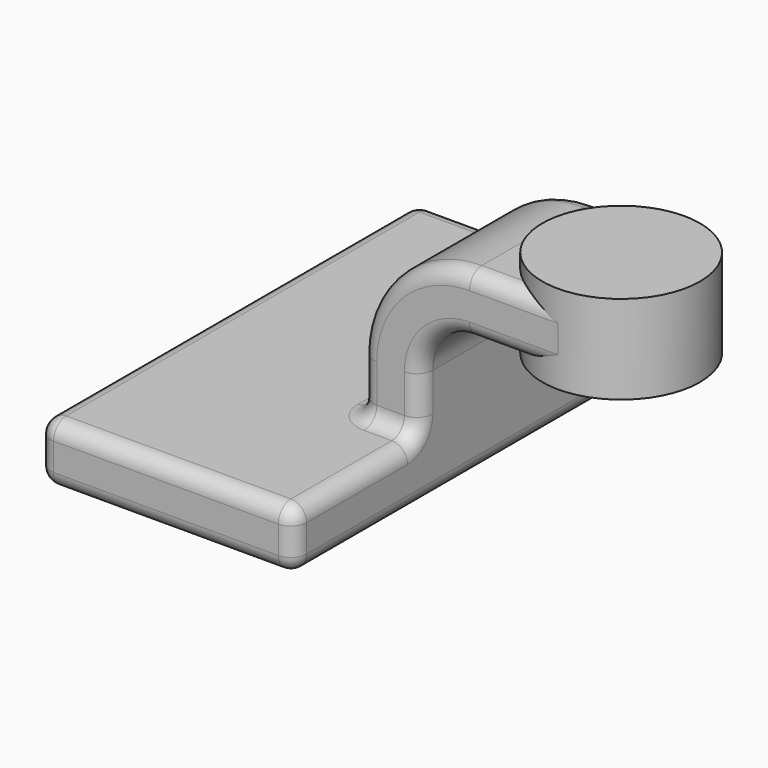
from build123d import *

# Parameters (mm, degrees)
F1_DEPTH      = 76.2
F0_W          = 25.4
F0_H          = 19.05
F2_DEPTH      = 25.4
F4_T1_DEPTH   = 142.24
F4_T3_DEPTH   = 90.17
F4_T5_DEPTH   = 17.4752
F4_T7_DEPTH   = 72.39
F4_T9_DEPTH   = 26.67
F4_T11_DEPTH  = 8.89
F4_S15_W      = 5.1816
F4_S15_H      = 5.1816
F4_T16_DEPTH  = 5.1816
F4_S21_W      = 5.1816
F4_S21_H      = 5.1816
F4_T22_DEPTH  = 5.1816
F4_S27_W      = 5.1816
F4_S27_H      = 5.1816
F4_T28_DEPTH  = 5.1816
F4_S33_W      = 5.1816
F4_S33_H      = 5.1816
F4_T34_DEPTH  = 5.1816
F4_S39_W      = 5.1816
F4_S39_H      = 5.1816
F4_T40_DEPTH  = 5.1816
F4_S45_W      = 5.1816
F4_S45_H      = 5.1816
F4_T46_DEPTH  = 5.1816
F4_T50_ANGLE  = 90
F4_T54_DEPTH  = 50.165
F4_S55_R      = 25.4
F4_T56_DEPTH  = 27
F4_T58_ANGLE  = 90
F4_T62_DEPTH  = 50.165
F4_S63_R      = 25.4
F4_T64_DEPTH  = 27
F4_T65_DEPTH  = 13.97
F4_T67_DEPTH  = 40.64
F4_T70_ANGLE  = 90
F4_T72_ANGLE  = 90
F4_T73_DEPTH  = 40.64
F4_T75_DEPTH  = 40.64
F4_T77_DEPTH  = 12.3952
F4_S81_W      = 5.1816
F4_S81_H      = 5.1816
F4_T82_DEPTH  = 5.1816
F4_S87_W      = 5.1816
F4_S87_H      = 5.1816
F4_T88_DEPTH  = 5.1816
F4_T92_ANGLE  = 90
F4_T96_DEPTH  = 50.165
F4_S97_R      = 25.4
F4_T98_DEPTH  = 27
F4_T100_ANGLE = 90
F4_T104_DEPTH = 50.165
F4_S105_R     = 25.4
F4_T106_DEPTH = 27
F4_T108_ANGLE = 90
F4_T110_ANGLE = 90


# Not quite as in the source:
# - a fillet or chamfer that OpenCascade refuses, or shapes differently, is made with other operations: its cross-section is extruded or revolved along the edge and cut away or added


with BuildPart() as f1:
    # F0 (on Front) → F1 (new body, symmetric)
    with BuildSketch(Plane.XZ):
        Polygon((-41.275, -9.525), (41.275, -9.525), (41.275, 9.525), (22.225, 9.525), (-41.275, 9.525), align=None)
    extrude(amount=F1_DEPTH, both=True)

    # F0 (on Front) → F2 (join, symmetric)
    with BuildSketch(Plane.XZ):
        with BuildLine():
            Line((22.225, 9.525), (41.275, 9.525))
            Line((41.275, 9.525), (41.275, 27.0002))
            ThreePointArc((41.275, 27.0002), (45.9246798487, 38.2255201513), (57.15, 42.8752))
            Line((57.15, 42.8752), (60.325, 42.8752))
            Line((60.325, 42.8752), (60.325, 61.9252))
            Line((60.325, 61.9252), (57.15, 61.9252))
            ThreePointArc((57.15, 61.9252), (32.4542956671, 51.6959043329), (22.225, 27.0002))
            Line((22.225, 27.0002), (22.225, 9.525))
        make_face()
        with Locations((73.025, 52.4002)):
            Rectangle(F0_W, F0_H)
    extrude(amount=F2_DEPTH, both=True)

    # F0 (on Front) → F3 (revolve)
    with BuildSketch(Plane.XZ):
        Polygon((85.725, 61.9252), (85.725, 42.8752), (85.725, 38.1), (111.125, 38.1), (111.125, 66.675), (85.725, 66.675), align=None)
    revolve(axis=Axis((85.725, 0, 52.3875), (0, 0, 1)))

    # F4: fillet of radius 5.08 on 31 edges, made by hand

    # F4_s2 → F4_t1 (cut)
    with BuildSketch(Plane.XZ.offset(-71.12)):
        with BuildLine():
            ThreePointArc((-41.275, 4.445), (-39.7871024484, 8.0371024484), (-36.195, 9.525))
            Line((-36.195, 9.525), (-41.275, 9.525))
            Line((-41.275, 9.525), (-41.275, 4.445))
        make_face()
        with BuildLine():
            ThreePointArc((-36.195, -9.525), (-39.7871024484, -8.0371024484), (-41.275, -4.445))
            Line((-41.275, -4.445), (-41.275, -9.525))
            Line((-41.275, -9.525), (-36.195, -9.525))
        make_face()
        with BuildLine():
            ThreePointArc((36.195, -9.525), (39.7871024484, -8.0371024484), (41.275, -4.445))
            Line((41.275, -4.445), (41.275, -9.525))
            Line((41.275, -9.525), (36.195, -9.525))
        make_face()
    extrude(amount=F4_T1_DEPTH, mode=Mode.SUBTRACT)

    # F4_s4 → F4_t3 (cut)
    with BuildSketch(Plane.YZ.offset(-36.195)):
        with BuildLine():
            ThreePointArc((76.2, 4.445), (74.7121024484, 8.0371024484), (71.12, 9.525))
            Line((71.12, 9.525), (76.2, 9.525))
            Line((76.2, 9.525), (76.2, 4.445))
        make_face()
        with BuildLine():
            ThreePointArc((-76.2, 4.445), (-74.7121024484, 8.0371024484), (-71.12, 9.525))
            Line((-71.12, 9.525), (-76.2, 9.525))
            Line((-76.2, 9.525), (-76.2, 4.445))
        make_face()
    extrude(amount=F4_T3_DEPTH, mode=Mode.SUBTRACT)

    # F4_s6 → F4_t5 (cut)
    with BuildSketch(Plane.XY.offset(9.525)):
        with BuildLine():
            ThreePointArc((27.305, -25.4), (23.7128975516, -23.9121024484), (22.225, -20.32))
            Line((22.225, -20.32), (22.225, -25.4))
            Line((22.225, -25.4), (27.305, -25.4))
        make_face()
        with BuildLine():
            ThreePointArc((27.305, 25.4), (23.7128975516, 23.9121024484), (22.225, 20.32))
            Line((22.225, 20.32), (22.225, 25.4))
            Line((22.225, 25.4), (27.305, 25.4))
        make_face()
    extrude(amount=F4_T5_DEPTH, mode=Mode.SUBTRACT)

    # F4_s8 → F4_t7 (cut)
    with BuildSketch(Plane.YZ.offset(-36.195)):
        with BuildLine():
            ThreePointArc((71.12, -9.525), (74.7121024484, -8.0371024484), (76.2, -4.445))
            Line((76.2, -4.445), (76.2, -9.525))
            Line((76.2, -9.525), (71.12, -9.525))
        make_face()
        with BuildLine():
            ThreePointArc((-71.12, -9.525), (-74.7121024484, -8.0371024484), (-76.2, -4.445))
            Line((-76.2, -4.445), (-76.2, -9.525))
            Line((-76.2, -9.525), (-71.12, -9.525))
        make_face()
    extrude(amount=F4_T7_DEPTH, mode=Mode.SUBTRACT)

    # F4_s10 → F4_t9 (cut)
    with BuildSketch(Plane.XY.offset(-4.445)):
        with BuildLine():
            ThreePointArc((36.195, 76.2), (39.7871024484, 74.7121024484), (41.275, 71.12))
            Line((41.275, 71.12), (41.275, 76.2))
            Line((41.275, 76.2), (36.195, 76.2))
        make_face()
        with BuildLine():
            ThreePointArc((41.275, -71.12), (39.7871024484, -74.7121024484), (36.195, -76.2))
            Line((36.195, -76.2), (41.275, -76.2))
            Line((41.275, -76.2), (41.275, -71.12))
        make_face()
    extrude(amount=F4_T9_DEPTH, mode=Mode.SUBTRACT)

    # F4_s12 → F4_t11 (cut)
    with BuildSketch(Plane.XY.offset(-4.445)):
        with BuildLine():
            ThreePointArc((-36.195, 76.2), (-39.7871024484, 74.7121024484), (-41.275, 71.12))
            Line((-41.275, 71.12), (-41.275, 76.2))
            Line((-41.275, 76.2), (-36.195, 76.2))
        make_face()
        with BuildLine():
            ThreePointArc((-36.195, -76.2), (-39.7871024484, -74.7121024484), (-41.275, -71.12))
            Line((-41.275, -71.12), (-41.275, -76.2))
            Line((-41.275, -76.2), (-36.195, -76.2))
        make_face()
    extrude(amount=F4_T11_DEPTH, mode=Mode.SUBTRACT)


with BuildPart() as f4_tool14:
    # F4_s15 → F4_t16 (new body)
    with BuildSketch(Plane.XZ.offset(71.12)):
        with Locations((-38.7858, 7.0358)):
            Rectangle(F4_S15_W, F4_S15_H)
    extrude(amount=F4_T16_DEPTH)

    # F4_s17 → F4_t18 (revolve, cut)
    with BuildSketch(Plane(origin=(-36.195, -71.12, 4.445), x_dir=(0.7071067812, 0, -0.7071067812), z_dir=(-0.7071067812, 0, -0.7071067812))):
        with BuildLine():
            ThreePointArc((0, -5.08), (5.08, 0), (0, 5.08))
            Line((0, 5.08), (0, -5.08))
        make_face()
    revolve(axis=Axis((-36.195, -71.12, 4.445), (0, -1, 0)), mode=Mode.SUBTRACT)


with BuildPart() as f1_1:
    add(f1.part)

    # F4_t13: cut F4_tool14
    add(f4_tool14.part, mode=Mode.SUBTRACT)


with BuildPart() as f4_tool20:
    # F4_s21 → F4_t22 (new body)
    with BuildSketch(Plane.XZ.offset(-71.12)):
        with Locations((-38.7858, 7.0358)):
            Rectangle(F4_S21_W, F4_S21_H)
    extrude(amount=-F4_T22_DEPTH)

    # F4_s23 → F4_t24 (revolve, cut)
    with BuildSketch(Plane(origin=(-36.195, 71.12, 4.445), x_dir=(0.7071067812, 0, -0.7071067812), z_dir=(0.7071067812, 0, 0.7071067812))):
        with BuildLine():
            ThreePointArc((0, -5.08), (5.08, 0), (0, 5.08))
            Line((0, 5.08), (0, -5.08))
        make_face()
    revolve(axis=Axis((-36.195, 71.12, 4.445), (0, 1, 0)), mode=Mode.SUBTRACT)


with BuildPart() as f1_2:
    add(f1_1.part)

    # F4_t19: cut F4_tool20
    add(f4_tool20.part, mode=Mode.SUBTRACT)


with BuildPart() as f4_tool26:
    # F4_s27 → F4_t28 (new body)
    with BuildSketch(Plane.XY.offset(-4.445)):
        with Locations((-38.7858, 73.7108)):
            Rectangle(F4_S27_W, F4_S27_H)
    extrude(amount=-F4_T28_DEPTH)

    # F4_s29 → F4_t30 (revolve, cut)
    with BuildSketch(Plane(origin=(-36.195, 71.12, -4.445), x_dir=(0.7071067812, -0.7071067812, 0), z_dir=(0.7071067812, 0.7071067812, 0))):
        with BuildLine():
            ThreePointArc((0, -5.08), (5.08, 0), (0, 5.08))
            Line((0, 5.08), (0, -5.08))
        make_face()
    revolve(axis=Axis((-36.195, 71.12, -4.445), (0, 0, -1)), mode=Mode.SUBTRACT)


with BuildPart() as f1_3:
    add(f1_2.part)

    # F4_t25: cut F4_tool26
    add(f4_tool26.part, mode=Mode.SUBTRACT)


with BuildPart() as f4_tool32:
    # F4_s33 → F4_t34 (new body)
    with BuildSketch(Plane.XY.offset(-4.445)):
        with Locations((38.7858, 73.7108)):
            Rectangle(F4_S33_W, F4_S33_H)
    extrude(amount=-F4_T34_DEPTH)

    # F4_s35 → F4_t36 (revolve, cut)
    with BuildSketch(Plane(origin=(36.195, 71.12, -4.445), x_dir=(-0.7071067812, -0.7071067812, 0), z_dir=(0.7071067812, -0.7071067812, 0))):
        with BuildLine():
            ThreePointArc((0, -5.08), (5.08, 0), (0, 5.08))
            Line((0, 5.08), (0, -5.08))
        make_face()
    revolve(axis=Axis((36.195, 71.12, -4.445), (0, 0, -1)), mode=Mode.SUBTRACT)


with BuildPart() as f1_4:
    add(f1_3.part)

    # F4_t31: cut F4_tool32
    add(f4_tool32.part, mode=Mode.SUBTRACT)


with BuildPart() as f4_tool38:
    # F4_s39 → F4_t40 (new body)
    with BuildSketch(Plane.XY.offset(-4.445)):
        with Locations((-38.7858, -73.7108)):
            Rectangle(F4_S39_W, F4_S39_H)
    extrude(amount=-F4_T40_DEPTH)

    # F4_s41 → F4_t42 (revolve, cut)
    with BuildSketch(Plane(origin=(-36.195, -71.12, -4.445), x_dir=(0.7071067812, 0.7071067812, 0), z_dir=(-0.7071067812, 0.7071067812, 0))):
        with BuildLine():
            ThreePointArc((0, -5.08), (5.08, 0), (0, 5.08))
            Line((0, 5.08), (0, -5.08))
        make_face()
    revolve(axis=Axis((-36.195, -71.12, -4.445), (0, 0, -1)), mode=Mode.SUBTRACT)


with BuildPart() as f1_5:
    add(f1_4.part)

    # F4_t37: cut F4_tool38
    add(f4_tool38.part, mode=Mode.SUBTRACT)


with BuildPart() as f4_tool44:
    # F4_s45 → F4_t46 (new body)
    with BuildSketch(Plane.XY.offset(-4.445)):
        with Locations((38.7858, -73.7108)):
            Rectangle(F4_S45_W, F4_S45_H)
    extrude(amount=-F4_T46_DEPTH)

    # F4_s47 → F4_t48 (revolve, cut)
    with BuildSketch(Plane(origin=(36.195, -71.12, -4.445), x_dir=(-0.7071067812, 0.7071067812, 0), z_dir=(-0.7071067812, -0.7071067812, 0))):
        with BuildLine():
            ThreePointArc((0, -5.08), (5.08, 0), (0, 5.08))
            Line((0, 5.08), (0, -5.08))
        make_face()
    revolve(axis=Axis((36.195, -71.12, -4.445), (0, 0, -1)), mode=Mode.SUBTRACT)


with BuildPart() as f1_6:
    add(f1_5.part)

    # F4_t43: cut F4_tool44
    add(f4_tool44.part, mode=Mode.SUBTRACT)

    # F4_s49 → F4_t50 (revolve, cut)
    with BuildSketch(Plane.YZ.offset(57.15)):
        with BuildLine():
            ThreePointArc((-25.4, 56.8452), (-23.9121024484, 60.4373024484), (-20.32, 61.9252))
            Line((-20.32, 61.9252), (-25.4, 61.9252))
            Line((-25.4, 61.9252), (-25.4, 56.8452))
        make_face()
    revolve(axis=Axis((57.15, -25.4, 27.0002), (0, -1, 0)), revolution_arc=F4_T50_ANGLE, mode=Mode.SUBTRACT)


with BuildPart() as f4_tool52:
    # F4_s53 → F4_t54 (new body)
    with BuildSketch(Plane.YZ.offset(107.315)):
        with BuildLine():
            ThreePointArc((-25.4, 56.8452), (-23.9121024484, 60.4373024484), (-20.32, 61.9252))
            Line((-20.32, 61.9252), (-25.4, 61.9252))
            Line((-25.4, 61.9252), (-25.4, 56.8452))
        make_face()
    extrude(amount=-F4_T54_DEPTH)

    # F4_s55 → F4_t56 (cut, symmetric)
    with BuildSketch(Plane.XY.offset(59.4)):
        with Locations((85.725, 0)):
            Circle(F4_S55_R)
    extrude(amount=F4_T56_DEPTH, both=True, mode=Mode.SUBTRACT)


with BuildPart() as f1_7:
    add(f1_6.part)

    # F4_t51: cut F4_tool52
    add(f4_tool52.part, mode=Mode.SUBTRACT)

    # F4_s57 → F4_t58 (revolve, cut)
    with BuildSketch(Plane.YZ.offset(57.15)):
        with BuildLine():
            ThreePointArc((25.4, 56.8452), (23.9121024484, 60.4373024484), (20.32, 61.9252))
            Line((20.32, 61.9252), (25.4, 61.9252))
            Line((25.4, 61.9252), (25.4, 56.8452))
        make_face()
    revolve(axis=Axis((57.15, 25.4, 27.0002), (0, -1, 0)), revolution_arc=F4_T58_ANGLE, mode=Mode.SUBTRACT)


with BuildPart() as f4_tool60:
    # F4_s61 → F4_t62 (new body)
    with BuildSketch(Plane.YZ.offset(107.315)):
        with BuildLine():
            ThreePointArc((25.4, 56.8452), (23.9121024484, 60.4373024484), (20.32, 61.9252))
            Line((20.32, 61.9252), (25.4, 61.9252))
            Line((25.4, 61.9252), (25.4, 56.8452))
        make_face()
    extrude(amount=-F4_T62_DEPTH)

    # F4_s63 → F4_t64 (cut, symmetric)
    with BuildSketch(Plane.XY.offset(59.4)):
        with Locations((85.725, 0)):
            Circle(F4_S63_R)
    extrude(amount=F4_T64_DEPTH, both=True, mode=Mode.SUBTRACT)


with BuildPart() as f1_8:
    add(f1_7.part)

    # F4_t59: cut F4_tool60
    add(f4_tool60.part, mode=Mode.SUBTRACT)

    # F4_s66 → F4_t65 (join)
    with BuildSketch(Plane.YZ.offset(27.305)):
        with BuildLine():
            ThreePointArc((30.48, 9.525), (26.8878975516, 11.0128975516), (25.4, 14.605))
            Line((25.4, 14.605), (25.4, 9.525))
            Line((25.4, 9.525), (30.48, 9.525))
        make_face()
        with BuildLine():
            ThreePointArc((-30.48, 9.525), (-26.8878975516, 11.0128975516), (-25.4, 14.605))
            Line((-25.4, 14.605), (-25.4, 9.525))
            Line((-25.4, 9.525), (-30.48, 9.525))
        make_face()
    extrude(amount=F4_T65_DEPTH)

    # F4_s68 → F4_t67 (join)
    with BuildSketch(Plane.XZ.offset(-20.32)):
        with BuildLine():
            ThreePointArc((17.145, 9.525), (20.7371024484, 11.0128975516), (22.225, 14.605))
            Line((22.225, 14.605), (22.225, 9.525))
            Line((22.225, 9.525), (17.145, 9.525))
        make_face()
    extrude(amount=F4_T67_DEPTH)

    # F4_s69 → F4_t70 (revolve)
    with BuildSketch(Plane.YZ.offset(27.305)):
        with BuildLine():
            ThreePointArc((-30.48, 9.525), (-26.8878975516, 11.0128975516), (-25.4, 14.605))
            Line((-25.4, 14.605), (-25.4, 9.525))
            Line((-25.4, 9.525), (-30.48, 9.525))
        make_face()
    revolve(axis=Axis((27.305, -20.32, 9.525), (0, 0, -1)), revolution_arc=F4_T70_ANGLE)

    # F4_s71 → F4_t72 (revolve)
    with BuildSketch(Plane.YZ.offset(27.305)):
        with BuildLine():
            ThreePointArc((30.48, 9.525), (26.8878975516, 11.0128975516), (25.4, 14.605))
            Line((25.4, 14.605), (25.4, 9.525))
            Line((25.4, 9.525), (30.48, 9.525))
        make_face()
    revolve(axis=Axis((27.305, 20.32, 9.525), (0, 0, 1)), revolution_arc=F4_T72_ANGLE)

    # F4_s74 → F4_t73 (cut)
    with BuildSketch(Plane.XZ.offset(-71.12)):
        with BuildLine():
            ThreePointArc((41.275, 4.445), (39.7871024484, 8.0371024484), (36.195, 9.525))
            Line((36.195, 9.525), (41.275, 9.525))
            Line((41.275, 9.525), (41.275, 4.445))
        make_face()
    extrude(amount=F4_T73_DEPTH, mode=Mode.SUBTRACT)

    # F4_s76 → F4_t75 (cut)
    with BuildSketch(Plane.XZ.offset(30.48)):
        with BuildLine():
            ThreePointArc((41.275, 4.445), (39.7871024484, 8.0371024484), (36.195, 9.525))
            Line((36.195, 9.525), (41.275, 9.525))
            Line((41.275, 9.525), (41.275, 4.445))
        make_face()
    extrude(amount=F4_T75_DEPTH, mode=Mode.SUBTRACT)

    # F4_s78 → F4_t77 (cut)
    with BuildSketch(Plane.XY.offset(14.605)):
        with BuildLine():
            ThreePointArc((41.275, -20.32), (39.7871024484, -23.9121024484), (36.195, -25.4))
            Line((36.195, -25.4), (41.275, -25.4))
            Line((41.275, -25.4), (41.275, -20.32))
        make_face()
        with BuildLine():
            ThreePointArc((41.275, 20.32), (39.7871024484, 23.9121024484), (36.195, 25.4))
            Line((36.195, 25.4), (41.275, 25.4))
            Line((41.275, 25.4), (41.275, 20.32))
        make_face()
    extrude(amount=F4_T77_DEPTH, mode=Mode.SUBTRACT)


with BuildPart() as f4_tool80:
    # F4_s81 → F4_t82 (new body)
    with BuildSketch(Plane.YZ.offset(36.195)):
        with Locations((-73.7108, 7.0358)):
            Rectangle(F4_S81_W, F4_S81_H)
    extrude(amount=F4_T82_DEPTH)

    # F4_s83 → F4_t84 (revolve, cut)
    with BuildSketch(Plane(origin=(36.195, -71.12, 4.445), x_dir=(0, 0.7071067812, -0.7071067812), z_dir=(0, -0.7071067812, -0.7071067812))):
        with BuildLine():
            ThreePointArc((0, -5.08), (5.08, 0), (0, 5.08))
            Line((0, 5.08), (0, -5.08))
        make_face()
    revolve(axis=Axis((36.195, -71.12, 4.445), (1, 0, 0)), mode=Mode.SUBTRACT)


with BuildPart() as f1_9:
    add(f1_8.part)

    # F4_t79: cut F4_tool80
    add(f4_tool80.part, mode=Mode.SUBTRACT)


with BuildPart() as f4_tool86:
    # F4_s87 → F4_t88 (new body)
    with BuildSketch(Plane.YZ.offset(36.195)):
        with Locations((73.7108, 7.0358)):
            Rectangle(F4_S87_W, F4_S87_H)
    extrude(amount=F4_T88_DEPTH)

    # F4_s89 → F4_t90 (revolve, cut)
    with BuildSketch(Plane(origin=(36.195, 71.12, 4.445), x_dir=(0, -0.7071067812, -0.7071067812), z_dir=(0, -0.7071067812, 0.7071067812))):
        with BuildLine():
            ThreePointArc((0, -5.08), (5.08, 0), (0, 5.08))
            Line((0, 5.08), (0, -5.08))
        make_face()
    revolve(axis=Axis((36.195, 71.12, 4.445), (1, 0, 0)), mode=Mode.SUBTRACT)


with BuildPart() as f1_10:
    add(f1_9.part)

    # F4_t85: cut F4_tool86
    add(f4_tool86.part, mode=Mode.SUBTRACT)

    # F4_s91 → F4_t92 (revolve, cut)
    with BuildSketch(Plane.XY.offset(27.0002)):
        with BuildLine():
            ThreePointArc((36.195, -25.4), (39.7871024484, -23.9121024484), (41.275, -20.32))
            Line((41.275, -20.32), (41.275, -25.4))
            Line((41.275, -25.4), (36.195, -25.4))
        make_face()
    revolve(axis=Axis((57.15, -25.4, 27.0002), (0, 1, 0)), revolution_arc=F4_T92_ANGLE, mode=Mode.SUBTRACT)


with BuildPart() as f4_tool94:
    # F4_s95 → F4_t96 (new body)
    with BuildSketch(Plane.YZ.offset(57.15)):
        with BuildLine():
            ThreePointArc((-25.4, 47.9552), (-23.9121024484, 44.3630975516), (-20.32, 42.8752))
            Line((-20.32, 42.8752), (-25.4, 42.8752))
            Line((-25.4, 42.8752), (-25.4, 47.9552))
        make_face()
    extrude(amount=F4_T96_DEPTH)

    # F4_s97 → F4_t98 (cut, symmetric)
    with BuildSketch(Plane.XY.offset(45.4)):
        with Locations((85.725, 0)):
            Circle(F4_S97_R)
    extrude(amount=F4_T98_DEPTH, both=True, mode=Mode.SUBTRACT)


with BuildPart() as f1_11:
    add(f1_10.part)

    # F4_t93: cut F4_tool94
    add(f4_tool94.part, mode=Mode.SUBTRACT)

    # F4_s99 → F4_t100 (revolve, cut)
    with BuildSketch(Plane.XY.offset(27.0002)):
        with BuildLine():
            ThreePointArc((41.275, 20.32), (39.7871024484, 23.9121024484), (36.195, 25.4))
            Line((36.195, 25.4), (41.275, 25.4))
            Line((41.275, 25.4), (41.275, 20.32))
        make_face()
    revolve(axis=Axis((57.15, 25.4, 27.0002), (0, 1, 0)), revolution_arc=F4_T100_ANGLE, mode=Mode.SUBTRACT)


with BuildPart() as f4_tool102:
    # F4_s103 → F4_t104 (new body)
    with BuildSketch(Plane.YZ.offset(57.15)):
        with BuildLine():
            ThreePointArc((25.4, 47.9552), (23.9121024484, 44.3630975516), (20.32, 42.8752))
            Line((20.32, 42.8752), (25.4, 42.8752))
            Line((25.4, 42.8752), (25.4, 47.9552))
        make_face()
    extrude(amount=F4_T104_DEPTH)

    # F4_s105 → F4_t106 (cut, symmetric)
    with BuildSketch(Plane.XY.offset(45.4)):
        with Locations((85.725, 0)):
            Circle(F4_S105_R)
    extrude(amount=F4_T106_DEPTH, both=True, mode=Mode.SUBTRACT)


with BuildPart() as f1_12:
    add(f1_11.part)

    # F4_t101: cut F4_tool102
    add(f4_tool102.part, mode=Mode.SUBTRACT)

    # F4_s107 → F4_t108 (revolve, cut)
    with BuildSketch(Plane.XZ.offset(-30.48)):
        with BuildLine():
            ThreePointArc((41.275, 4.445), (39.7871024484, 8.0371024484), (36.195, 9.525))
            Line((36.195, 9.525), (41.275, 9.525))
            Line((41.275, 9.525), (41.275, 4.445))
        make_face()
    revolve(axis=Axis((41.275, 30.48, 14.605), (-1, 0, 0)), revolution_arc=F4_T108_ANGLE, mode=Mode.SUBTRACT)

    # F4_s109 → F4_t110 (revolve, cut)
    with BuildSketch(Plane.XZ.offset(30.48)):
        with BuildLine():
            ThreePointArc((41.275, 4.445), (39.7871024484, 8.0371024484), (36.195, 9.525))
            Line((36.195, 9.525), (41.275, 9.525))
            Line((41.275, 9.525), (41.275, 4.445))
        make_face()
    revolve(axis=Axis((41.275, -30.48, 14.605), (1, 0, 0)), revolution_arc=F4_T110_ANGLE, mode=Mode.SUBTRACT)


solid = f1_12.part
